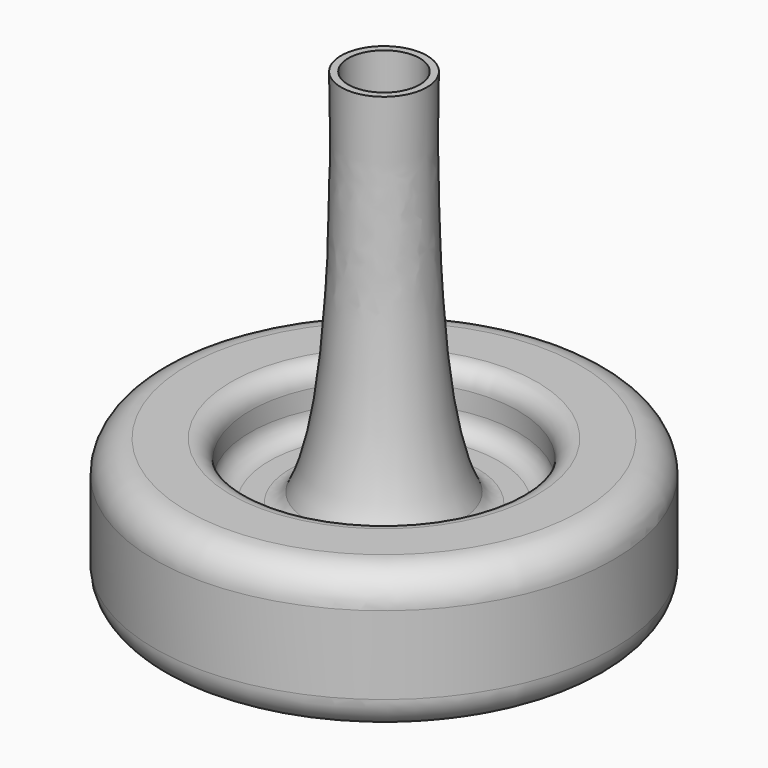
from build123d import *

# Parameters (mm, degrees)
F2_R     = 4.7625
F4_DEPTH = 9.525
F5_R     = 1.27
F6_DEPTH = 10.16
F8_R     = 7.62
F9_R     = 4.318
F10_R    = 2.54
F11_R    = 2.54


# Not quite as in the source:
# - a fillet or chamfer that OpenCascade refuses, or shapes differently, is made with other operations: its cross-section is extruded or revolved along the edge and cut away or added


with BuildPart() as f1:
    # F0 (on Front) → F1 (revolve)
    with BuildSketch(Plane.XZ):
        with BuildLine():
            Line((30.5308, 1.4264921218), (30.5308, 20.4764921218))
            Line((30.5308, 20.4764921218), (17.8308, 20.4764921218))
            Line((17.8308, 20.4764921218), (17.8308, 12.8564921218))
            Line((17.8308, 12.8564921218), (11.0718724159, 12.8564921218))
            add(Edge.make_bspline(
                [(5.715, 63.5), (5.5530331762, 56.4786912002), (5.6875657666, 53.6654097305), (6.2509646676, 19.2247689696), (11.0718724159, 12.8564921218)],
                knots=[0, 0, 0, 0, 0.3762820924, 1, 1, 1, 1], degree=3))
            Line((5.715, 63.5), (0, 63.5))
            Line((0, 63.5), (0, 0))
            Line((0, 0), (2.54, 0))
            Line((2.54, 0), (5.1308, 9.0464921218))
            Line((5.1308, 9.0464921218), (17.8308, 9.0464921218))
            Line((17.8308, 9.0464921218), (17.8308, 1.4264921218))
            Line((17.8308, 1.4264921218), (30.5308, 1.4264921218))
        make_face()
    revolve(axis=Axis((0, 0, 31.75), (0, 0, -1)))

    # F2 (on face) → F4 (cut)
    with BuildSketch(Plane.XY.offset(63.5)):
        Circle(F2_R)
    extrude(amount=-F4_DEPTH, mode=Mode.SUBTRACT)

    # F5 (on face) → F6 (cut)
    with BuildSketch(Plane(origin=(0, 0, 0), x_dir=(1, 0, 0), z_dir=(0, 0, -1))):
        Circle(F5_R)
    extrude(amount=-F6_DEPTH, mode=Mode.SUBTRACT)

    # F7: fillet of radius 2.54 on 1 edges, made by hand

    # F7_s1 → F7_t2 (revolve, cut)
    with BuildSketch(Plane.XZ):
        with BuildLine():
            ThreePointArc((3.0413485481, 1.7505966073), (2.3849498356, 0.6433048613), (1.27, 0))
            Line((1.27, 0), (2.54, 0))
            Line((2.54, 0), (3.0413485481, 1.7505966073))
        make_face()
    revolve(axis=Axis((0, 0, 0), (0, 0, -1)), mode=Mode.SUBTRACT)

    # F8
    f8_edges = [f1.edges().sort_by_distance(p)[0] for p in [
        (-5.1308, 0, 9.046492),
    ]]
    fillet(f8_edges, radius=F8_R)

    # F9
    f9_edges = [f1.edges().sort_by_distance(p)[0] for p in [
        (-30.5308, 0, 1.426492),
        (-30.5308, 0, 20.476492),
        (30.5308, 0, 10.951492),
    ]]
    fillet(f9_edges, radius=F9_R)

    # F10
    f10_edges = [f1.edges().sort_by_distance(p)[0] for p in [
        (-11.071872, 0, 12.856492),
        (-17.8308, 0, 12.856492),
        (-17.8308, 0, 20.476492),
        (17.8308, 0, 16.666492),
    ]]
    fillet(f10_edges, radius=F10_R)

    # F11
    f11_edges = [f1.edges().sort_by_distance(p)[0] for p in [
        (-17.8308, 0, 9.046492),
        (-17.8308, 0, 1.426492),
        (17.8308, 0, 5.236492),
    ]]
    fillet(f11_edges, radius=F11_R)


solid = f1.part
